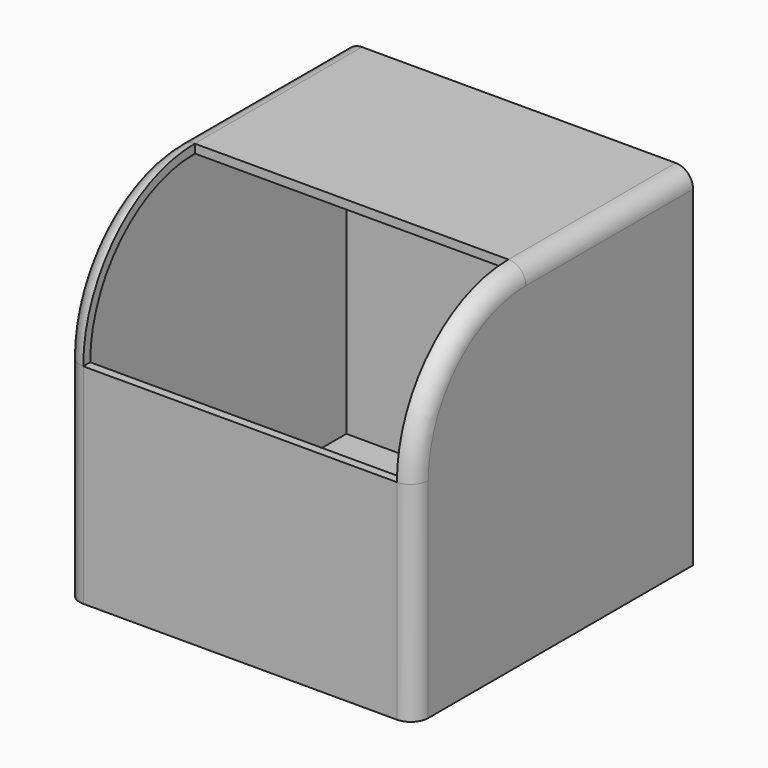
from build123d import *

# Parameters (mm, degrees)
F0_W     = 100
F0_H     = 100
F1_DEPTH = 100
F2_R     = 40
F3_R     = 5
F4_T     = 2.5


# Not quite as in the source:
# - a shell that OpenCascade refuses in one call is made with other operations: the cavity is built on its own and cut out


with BuildPart() as f1:
    # F0 (on Top) → F1 (new body)
    with BuildSketch(Plane.XY):
        Rectangle(F0_W, F0_H)
    extrude(amount=F1_DEPTH)

    # F2
    f2_edges = [f1.edges().sort_by_distance(p)[0] for p in [
        (0, -50, 100),
    ]]
    fillet(f2_edges, radius=F2_R)

    # F3
    f3_edges = [f1.edges().sort_by_distance(p)[0] for p in [
        (50, 20, 100),
        (-50, 20, 100),
    ]]
    fillet(f3_edges, radius=F3_R)

    # F4: shell of thickness 2.5, made by hand


with BuildPart() as f4_core1:
    # F4_t2: copy of F1
    add(f1.part)

    # the walls: a layer under each face that stays
    f4_faces = [f4_core1.faces().sort_by_distance(p)[0] for p in [
        (0, -50, 30),
        (-48.5355339059, -48.5355339059, 30),
        (48.5355339059, -48.5355339059, 30),
        (0, 0, 0),
        (-48.5355339059, -37.2487373415, 87.2487373415),
        (48.5355339059, -37.2487373415, 87.2487373415),
        (0, 20, 100),
        (-50, 2.5, 47.5),
        (50, 2.5, 47.5),
        (0, 50, 50),
        (-48.5355339059, 20, 98.5355339059),
        (48.5355339059, 20, 98.5355339059),
    ]]
    thicken(f4_faces, amount=-F4_T, mode=Mode.SUBTRACT)


with BuildPart() as f1_1:
    add(f1.part)

    # what is left inside the walls is the cavity
    f4_cavity = [f4_core1.part.solids().sort_by_distance(p)[0] for p in [
        (0, -15.833333, 2.525),
    ]]
    add(f4_cavity, mode=Mode.SUBTRACT)


solid = f1_1.part
